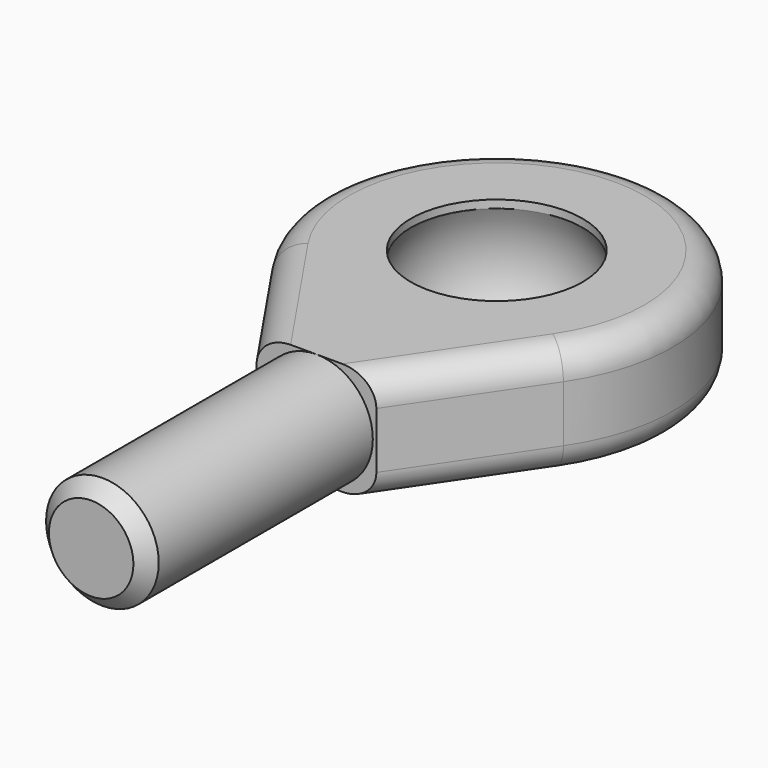
from build123d import *

# Parameters (mm, degrees)
F0_R     = 154.94
F1_DEPTH = 203.2
F3_DEPTH = 508
F6_R     = 50.8


# Not quite as in the source:
# - a fillet or chamfer that OpenCascade refuses, or shapes differently, is made with other operations: its cross-section is extruded or revolved along the edge and cut away or added


with BuildPart() as f1:
    # F0 (on Top) → F1 (new body)
    with BuildSketch(Plane.XY):
        with BuildLine():
            Line((107.95, -406.4), (262.736611536, -178.2574625608))
            ThreePointArc((262.736611536, -178.2574625608), (0, 317.5), (-262.736611536, -178.2574625608))
            Line((-262.736611536, -178.2574625608), (-107.95, -406.4))
            Line((-107.95, -406.4), (0, -406.4))
            Line((0, -406.4), (107.95, -406.4))
        make_face()
        Circle(F0_R, mode=Mode.SUBTRACT)
    extrude(amount=F1_DEPTH)

    # F2 (on face) → F3 (join)
    with BuildSketch(Plane.XZ.offset(406.4)):
        with BuildLine():
            ThreePointArc((-6.5e-08, 0), (71.8420489456, 29.7579510085), (101.6, 101.6))
            ThreePointArc((101.6, 101.6), (71.8420489961, 173.442048941), (7.8e-08, 203.2))
            ThreePointArc((7.8e-08, 203.2), (-101.6, 101.6000000715), (-6.5e-08, 0))
        make_face()
    extrude(amount=F3_DEPTH)

    # F4 (on Right) → F5 (revolve, cut)
    with BuildSketch(Plane.YZ):
        with BuildLine():
            Line((0, 203.2), (-145.9118912221, 203.2))
            ThreePointArc((-145.9118912221, 203.2), (-177.8, 101.6), (-145.9118912221, 0))
            Line((-145.9118912221, 0), (0, 0))
            Line((0, 0), (0, 203.2))
        make_face()
    revolve(axis=Axis((0, 0, 101.6), (0, 0, -1)), mode=Mode.SUBTRACT)

    # F6
    f6_edges = [f1.edges().sort_by_distance(p)[0] for p in [
        (262.736612, -178.257463, 101.6),
        (-262.736612, -178.257463, 101.6),
        (0, 317.5, 0),
        (0, 317.5, 203.2),
        (-185.343306, -292.328731, 0),
        (-185.343306, -292.328731, 203.2),
        (185.343306, -292.328731, 0),
        (185.343306, -292.328731, 203.2),
    ]]
    fillet(f6_edges, radius=F6_R)

    # F7: chamfer of 25.4 on 1 edges, made by hand

    # F7_s1 → F7_t2 (revolve, cut)
    with BuildSketch(Plane.YZ):
        Polygon((-889, 0), (-914.4, 25.4), (-914.4, 0), align=None)
    revolve(axis=Axis((0, -914.4, 101.6), (0, 1, 0)), mode=Mode.SUBTRACT)


solid = f1.part
